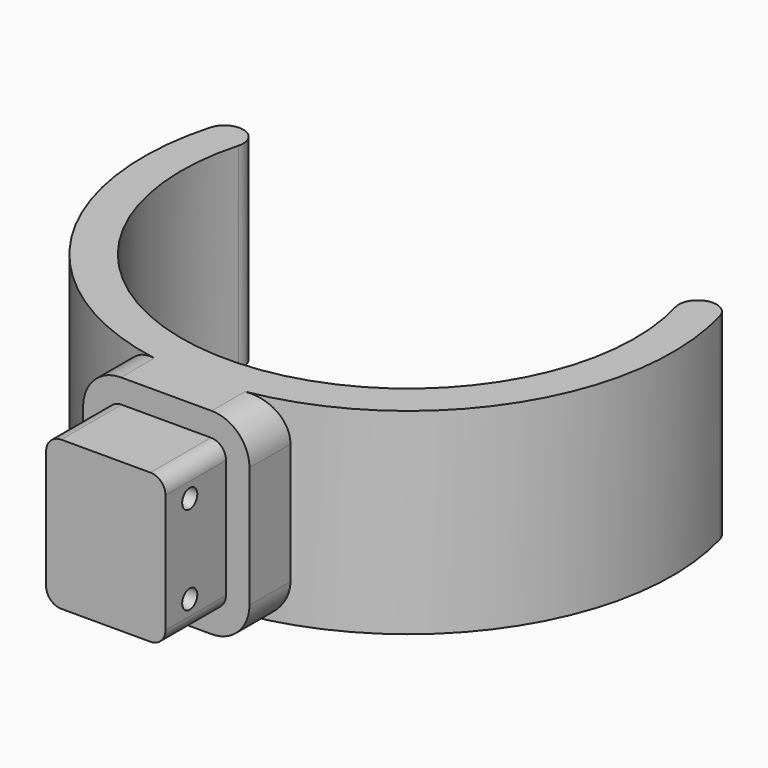
from build123d import *

# Parameters (mm, degrees)
F0_W          = 5
F0_H          = 26
F1_ANGLE_BACK = 110
F1_ANGLE      = 220
F2_W          = 22
F2_H          = 26
F3_DEPTH      = 5
F3_DEPTH_BACK = 5
F4_R          = 2.49999
F5_W          = 15.8
F5_H          = 19.7
F6_DEPTH      = 10
F7_R          = 1.25
F8_DEPTH      = 42.901
F9_R          = 2
F10_R         = 5


# Not quite as in the source:
# - a fillet or chamfer is up to 0.001 mm smaller than in the source, because OpenCascade refuses the exact size


with BuildPart() as f1:
    # F0 (on Right) → F1 (revolve)
    with BuildSketch(Plane.YZ, mode=Mode.PRIVATE) as f1_sk:
        with Locations((2.5, 0)):
            Rectangle(F0_W, F0_H)
    revolve(f1_sk.sketch.rotate(Axis((0, 35, 2.8591789305), (0, 0, -1)), -F1_ANGLE_BACK), axis=Axis((0, 35, 2.8591789305), (0, 0, -1)), revolution_arc=F1_ANGLE)

    # F2 (on Front) → F3 (join, two sides)
    with BuildSketch(Plane.XZ) as f3_sk:
        Rectangle(F2_W, F2_H)
    extrude(amount=F3_DEPTH)
    extrude(f3_sk.sketch, amount=-F3_DEPTH_BACK)

    # F4 (radius 2.5 in the source; OpenCascade refuses exactly that, so slightly less here)
    f4_edges = [f1.edges().sort_by_distance(p)[0] for p in [
        (32.889242, 46.970705, 0),
        (28.190779, 45.260604, 0),
        (-28.190779, 45.260604, 0),
        (-32.889242, 46.970705, 0),
    ]]
    fillet(f4_edges, radius=F4_R)

    # F5 (on face) → F6 (join)
    with BuildSketch(Plane.XZ.offset(5)):
        Rectangle(F5_W, F5_H)
    extrude(amount=F6_DEPTH)

    # F7 (on face) → F8 (cut, through all)
    with BuildSketch(Plane.YZ.offset(7.9)):
        with Locations((-11, 5.85)):
            Circle(F7_R)
        with Locations((-11, -5.85)):
            Circle(F7_R)
    extrude(amount=-F8_DEPTH, mode=Mode.SUBTRACT)

    # F9
    f9_edges = [f1.edges().sort_by_distance(p)[0] for p in [
        (7.9, -10, 9.85),
        (7.9, -10, -9.85),
        (-7.9, -10, -9.85),
        (-7.9, -10, 9.85),
    ]]
    fillet(f9_edges, radius=F9_R)

    # F10
    f10_edges = [f1.edges().sort_by_distance(p)[0] for p in [
        (-11, -1.613248, 13),
        (-11, -1.613248, -13),
        (11, -1.613248, -13),
        (11, -1.613248, 13),
    ]]
    fillet(f10_edges, radius=F10_R)


solid = f1.part
